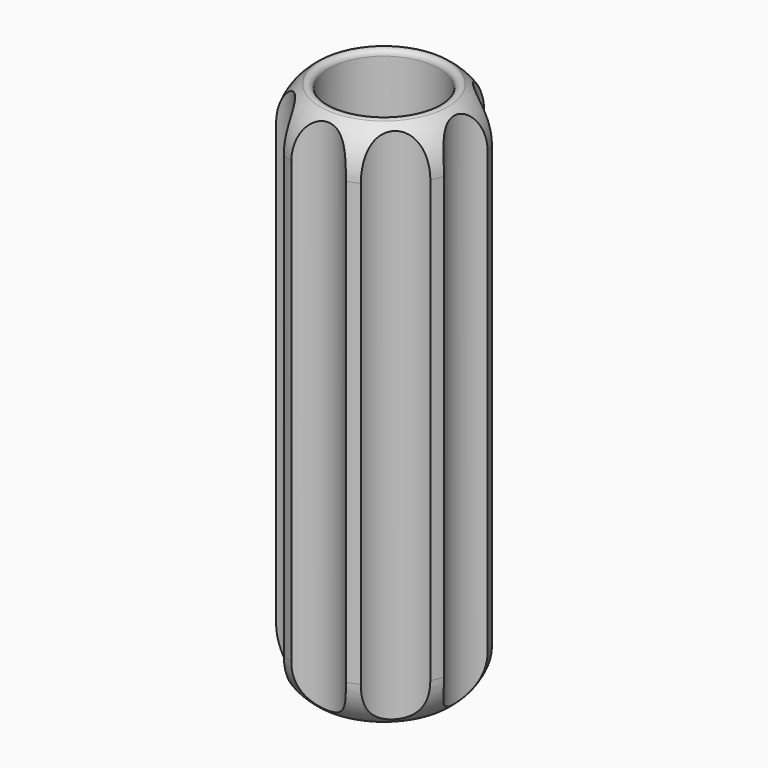
from build123d import *

# Parameters (mm, degrees)
F3_R     = 3.5
F4_DEPTH = 100
F5_R     = 0.5


# Not quite as in the source:
# - a fillet or chamfer that OpenCascade refuses, or shapes differently, is made with other operations: its cross-section is extruded or revolved along the edge and cut away or added
# - a feature names something its author has since deleted; it is built from what else it names


with BuildPart() as f1:
    # F0 (on Front) → F1 (revolve)
    with BuildSketch(Plane.XZ):
        Polygon((-5.1, 35), (-5.1, 50), (-8, 50), (-8, 0), (-5.1, 0), (-5.1, 33), (0, 33), (0, 35), align=None)
    revolve(axis=Axis((0, 0, 34), (0, 0, -1)))

    # F2: fillet of radius 5 on 2 edges, made by hand

    # F2_s1 → F2_t2 (revolve, cut)
    with BuildSketch(Plane.XZ):
        with BuildLine():
            ThreePointArc((-5.1, 50), (-7.2130748866, 48.1549618818), (-8, 45.4623794782))
            Line((-8, 45.4623794782), (-8, 50))
            Line((-8, 50), (-5.1, 50))
        make_face()
    revolve(axis=Axis((0, 0, 50), (0, 0, -1)), mode=Mode.SUBTRACT)

    # F2_s3 → F2_t4 (revolve, cut)
    with BuildSketch(Plane.XZ):
        with BuildLine():
            ThreePointArc((-8, 4.5376205218), (-7.2130748866, 1.8450381182), (-5.1, 0))
            Line((-5.1, 0), (-8, 0))
            Line((-8, 0), (-8, 4.5376205218))
        make_face()
    revolve(axis=Axis((0, 0, 0), (0, 0, -1)), mode=Mode.SUBTRACT)

    # F3 (on Top) → F4 (cut)
    with BuildSketch(Plane.XY):
        with Locations((0, 10)):
            Circle(F3_R)
        with Locations((7.0710678119, 7.0710678119)):
            Circle(F3_R)
        with Locations((10, 0)):
            Circle(F3_R)
        with Locations((7.0710678119, -7.0710678119)):
            Circle(F3_R)
        with Locations((0, -10)):
            Circle(F3_R)
        with Locations((-7.0710678119, -7.0710678119)):
            Circle(F3_R)
        with Locations((-10, 0)):
            Circle(F3_R)
        with Locations((-7.0710678119, 7.0710678119)):
            Circle(F3_R)
    extrude(amount=F4_DEPTH, mode=Mode.SUBTRACT)

    # F5
    f5_edges = [f1.edges().sort_by_distance(p)[0] for p in [
        (5.1, 0, 50),
        (5.1, 0, 0),
    ]]
    fillet(f5_edges, radius=F5_R)


solid = f1.part
